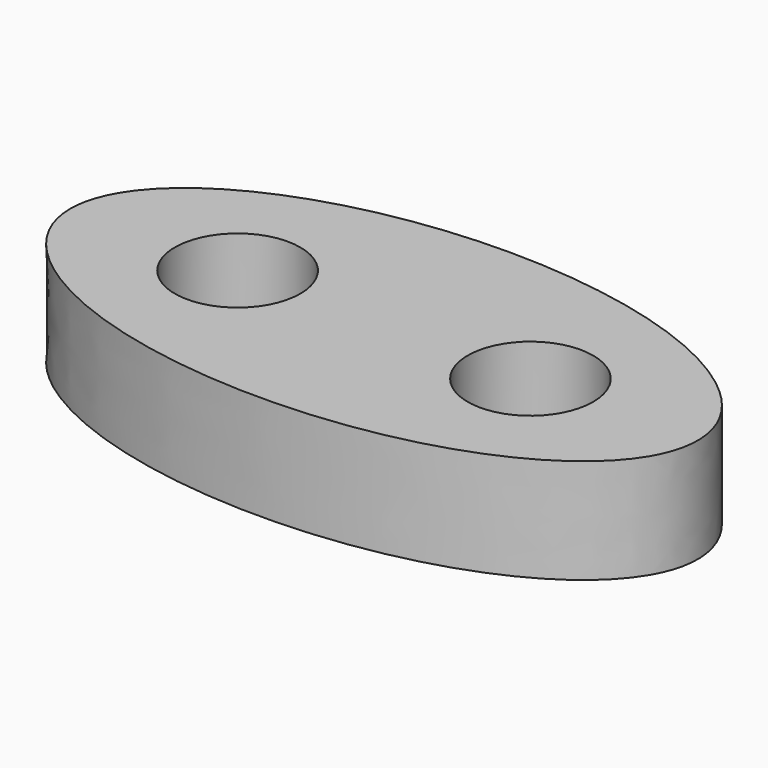
from build123d import *

# Parameters (mm, degrees)
F0_R     = 3
F1_DEPTH = 5


# Not quite as in the source:
# - a feature names something its author has since deleted; it is built from what else it names


with BuildPart() as f1:
    # F0 (on Top) → F1 (new body)
    with BuildSketch(Plane.XY):
        with BuildLine():
            add(Edge.make_bspline(
                [(-15, 0), (-15, -12.9903810568), (7.5, -6.4951905284), (30, 0), (7.5, 6.4951905284), (-15, 12.9903810568), (-15, 0)],
                knots=[0, 0, 0, 2.0943951024, 2.0943951024, 4.1887902048, 4.1887902048, 6.2831853072, 6.2831853072, 6.2831853072], degree=2, weights=[1, 0.5, 1, 0.5, 1, 0.5, 1]))
        make_face()
        with Locations((-7, 0)):
            Circle(F0_R, mode=Mode.SUBTRACT)
        with Locations((7, 0)):
            Circle(F0_R, mode=Mode.SUBTRACT)
    extrude(amount=F1_DEPTH)


solid = f1.part
